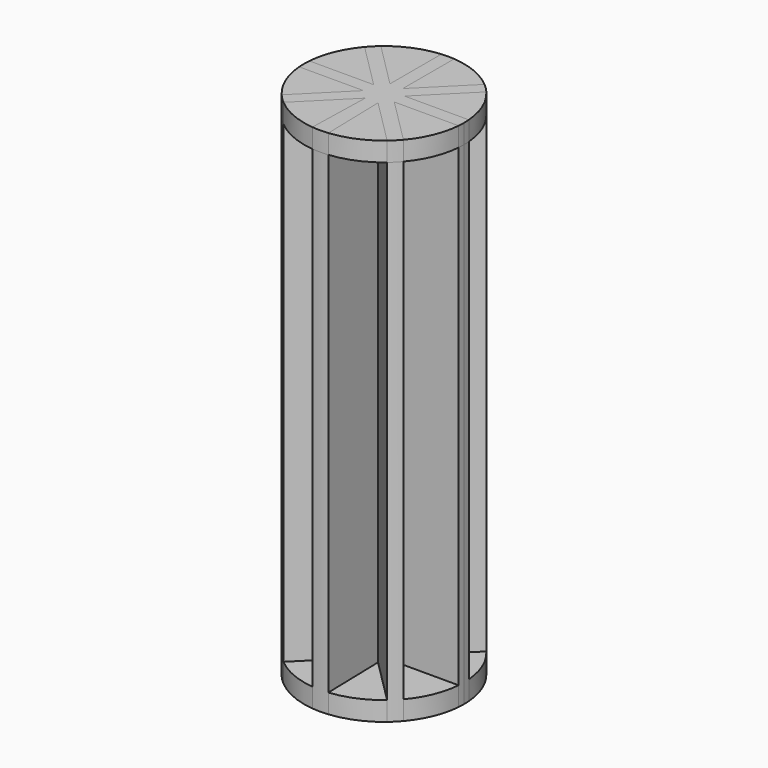
from build123d import *
from build123d import SkipClean  # not in build123d's __all__

# Parameters (mm, degrees)
F1_DEPTH = 3
F2_DEPTH = 80
F4_DEPTH = 3


with BuildPart() as f1:
    # F0 (on Top) → F1 (new body)
    with BuildSketch(Plane.XY):
        with BuildLine():
            Line((1, 2.4142135624), (8.1033983122, 9.5176118745))
            ThreePointArc((8.1033983122, 9.5176118745), (4.7835429046, 11.5484941564), (1, 12.4599357944))
            Line((1, 12.4599357944), (1, 2.4142135624))
        make_face()
    extrude(amount=F1_DEPTH)



with BuildPart() as f1b:
    # F0 (on Top) → F1, piece 2 (new body)
    with BuildSketch(Plane.XY):
        with BuildLine():
            Line((-1, 2.4142135624), (-1, 12.4599357944))
            ThreePointArc((-1, 12.4599357944), (-4.7835429046, 11.5484941564), (-8.1033983122, 9.5176118745))
            Line((-8.1033983122, 9.5176118745), (-1, 2.4142135624))
        make_face()
    extrude(amount=F1_DEPTH)


with BuildPart() as f1c:
    # F0 (on Top) → F1, piece 3 (new body)
    with BuildSketch(Plane.XY):
        with BuildLine():
            Line((2.4142135624, 1), (12.4599357944, 1))
            ThreePointArc((12.4599357944, 1), (11.5484941564, 4.7835429046), (9.5176118745, 8.1033983122))
            Line((9.5176118745, 8.1033983122), (2.4142135624, 1))
        make_face()
    extrude(amount=F1_DEPTH)


with BuildPart() as f1d:
    # F0 (on Top) → F1, piece 4 (new body)
    with BuildSketch(Plane.XY):
        with BuildLine():
            ThreePointArc((9.5176118745, -8.1033983122), (11.5484941564, -4.7835429046), (12.4599357944, -1))
            Line((12.4599357944, -1), (2.4142135624, -1))
            Line((2.4142135624, -1), (9.5176118745, -8.1033983122))
        make_face()
    extrude(amount=F1_DEPTH)


with BuildPart() as f1e:
    # F0 (on Top) → F1, piece 5 (new body)
    with BuildSketch(Plane.XY):
        with BuildLine():
            Line((-12.4599357944, 1), (-2.4142135624, 1))
            Line((-2.4142135624, 1), (-9.5176118745, 8.1033983122))
            ThreePointArc((-9.5176118745, 8.1033983122), (-11.5484941564, 4.7835429046), (-12.4599357944, 1))
        make_face()
    extrude(amount=F1_DEPTH)


with BuildPart() as f1f:
    # F0 (on Top) → F1, piece 6 (new body)
    with BuildSketch(Plane.XY):
        with BuildLine():
            ThreePointArc((-12.4599357944, -1), (-11.5484941564, -4.7835429046), (-9.5176118745, -8.1033983122))
            Line((-9.5176118745, -8.1033983122), (-2.4142135624, -1))
            Line((-2.4142135624, -1), (-12.4599357944, -1))
        make_face()
    extrude(amount=F1_DEPTH)


with BuildPart() as f1g:
    # F0 (on Top) → F1, piece 7 (new body)
    with BuildSketch(Plane.XY):
        with BuildLine():
            ThreePointArc((-8.1033983122, -9.5176118745), (-4.899257332, -11.499881634), (-1.25, -12.4373429638))
            Line((-1.25, -12.4373429638), (-1, -2.4142135624))
            Line((-1, -2.4142135624), (-8.1033983122, -9.5176118745))
        make_face()
    extrude(amount=F1_DEPTH)


with BuildPart() as f1h:
    # F0 (on Top) → F1, piece 8 (new body)
    with BuildSketch(Plane.XY):
        with BuildLine():
            ThreePointArc((1.25, -12.4373429638), (4.899257332, -11.499881634), (8.1033983122, -9.5176118745))
            Line((8.1033983122, -9.5176118745), (1, -2.4142135624))
            Line((1, -2.4142135624), (1.25, -12.4373429638))
        make_face()
    extrude(amount=F1_DEPTH)


with BuildPart() as f1_1:
    add(f1.part, clean=False)

    add(f1b.part)  # F2 merges F1b

    add(f1c.part)  # F2 merges F1c

    add(f1d.part)  # F2 merges F1d

    add(f1e.part)  # F2 merges F1e

    add(f1f.part)  # F2 merges F1f

    add(f1g.part)  # F2 merges F1g

    add(f1h.part)  # F2 merges F1h
    # F0 (on Top) → F2 (join)
    with BuildSketch(Plane.XY):
        with BuildLine():
            Line((1, 2.4142135624), (1, 12.4599357944))
            ThreePointArc((1, 12.4599357944), (0, 12.5), (-1, 12.4599357944))
            Line((-1, 12.4599357944), (-1, 2.4142135624))
            Line((-1, 2.4142135624), (0, 1.4142135624))
            Line((0, 1.4142135624), (1, 2.4142135624))
        make_face()
        with BuildLine():
            Line((2.4142135624, 1), (9.5176118745, 8.1033983122))
            ThreePointArc((9.5176118745, 8.1033983122), (8.8388347648, 8.8388347648), (8.1033983122, 9.5176118745))
            Line((8.1033983122, 9.5176118745), (1, 2.4142135624))
            Line((1, 2.4142135624), (0, 1.4142135624))
            Line((0, 1.4142135624), (-1, 2.4142135624))
            Line((-1, 2.4142135624), (-8.1033983122, 9.5176118745))
            ThreePointArc((-8.1033983122, 9.5176118745), (-8.8388347648, 8.8388347648), (-9.5176118745, 8.1033983122))
            Line((-9.5176118745, 8.1033983122), (-2.4142135624, 1))
            Line((-2.4142135624, 1), (0, -1.4142135624))
            Line((0, -1.4142135624), (1, -2.4142135624))
            Line((1, -2.4142135624), (8.1033983122, -9.5176118745))
            ThreePointArc((8.1033983122, -9.5176118745), (8.8388347648, -8.8388347648), (9.5176118745, -8.1033983122))
            Line((9.5176118745, -8.1033983122), (2.4142135624, -1))
            Line((2.4142135624, -1), (1.4142135624, 0))
            Line((1.4142135624, 0), (2.4142135624, 1))
        make_face()
        with BuildLine():
            Line((-1, -2.4142135624), (0, -1.4142135624))
            Line((0, -1.4142135624), (-2.4142135624, 1))
            Line((-2.4142135624, 1), (-12.4599357944, 1))
            ThreePointArc((-12.4599357944, 1), (-12.5, 0), (-12.4599357944, -1))
            Line((-12.4599357944, -1), (-2.4142135624, -1))
            Line((-2.4142135624, -1), (-9.5176118745, -8.1033983122))
            ThreePointArc((-9.5176118745, -8.1033983122), (-8.8388347648, -8.8388347648), (-8.1033983122, -9.5176118745))
            Line((-8.1033983122, -9.5176118745), (-1, -2.4142135624))
        make_face()
        with BuildLine():
            ThreePointArc((12.4599357944, -1), (12.4899799325, -0.5004011242), (12.5, 0))
            ThreePointArc((12.5, 0), (12.4899799325, 0.5004011242), (12.4599357944, 1))
            Line((12.4599357944, 1), (2.4142135624, 1))
            Line((2.4142135624, 1), (1.4142135624, 0))
            Line((1.4142135624, 0), (2.4142135624, -1))
            Line((2.4142135624, -1), (12.4599357944, -1))
        make_face()
        with BuildLine():
            ThreePointArc((-1.25, -12.4373429638), (0, -12.5), (1.25, -12.4373429638))
            Line((1.25, -12.4373429638), (1, -2.4142135624))
            Line((1, -2.4142135624), (0, -1.4142135624))
            Line((0, -1.4142135624), (-1, -2.4142135624))
            Line((-1, -2.4142135624), (-1.25, -12.4373429638))
        make_face()
    extrude(amount=F2_DEPTH)

    # F3 (on face) → F4 (join)
    with BuildSketch(Plane.XY.offset(80)):
        with BuildLine():
            Line((1, 2.4142135624), (8.1033983122, 9.5176118745))
            ThreePointArc((8.1033983122, 9.5176118745), (4.7835429046, 11.5484941564), (1, 12.4599357944))
            Line((1, 12.4599357944), (1, 2.4142135624))
        make_face()
        with BuildLine():
            Line((-1, 2.4142135624), (-1, 12.4599357944))
            ThreePointArc((-1, 12.4599357944), (-4.7835429046, 11.5484941564), (-8.1033983122, 9.5176118745))
            Line((-8.1033983122, 9.5176118745), (-1, 2.4142135624))
        make_face()
        with BuildLine():
            ThreePointArc((12.4599357944, -1), (12.4899799325, -0.5004011242), (12.5, 0))
            ThreePointArc((12.5, 0), (12.4899799325, 0.5004011242), (12.4599357944, 1))
            Line((12.4599357944, 1), (2.4142135624, 1))
            Line((2.4142135624, 1), (9.5176118745, 8.1033983122))
            ThreePointArc((9.5176118745, 8.1033983122), (8.8388347648, 8.8388347648), (8.1033983122, 9.5176118745))
            Line((8.1033983122, 9.5176118745), (1, 2.4142135624))
            Line((1, 2.4142135624), (1, 12.4599357944))
            ThreePointArc((1, 12.4599357944), (0, 12.5), (-1, 12.4599357944))
            Line((-1, 12.4599357944), (-1, 2.4142135624))
            Line((-1, 2.4142135624), (-8.1033983122, 9.5176118745))
            ThreePointArc((-8.1033983122, 9.5176118745), (-8.8388347648, 8.8388347648), (-9.5176118745, 8.1033983122))
            Line((-9.5176118745, 8.1033983122), (-2.4142135624, 1))
            Line((-2.4142135624, 1), (-12.4599357944, 1))
            ThreePointArc((-12.4599357944, 1), (-12.5, 0), (-12.4599357944, -1))
            Line((-12.4599357944, -1), (-2.4142135624, -1))
            Line((-2.4142135624, -1), (-9.5176118745, -8.1033983122))
            ThreePointArc((-9.5176118745, -8.1033983122), (-8.8388347648, -8.8388347648), (-8.1033983122, -9.5176118745))
            Line((-8.1033983122, -9.5176118745), (-1, -2.4142135624))
            Line((-1, -2.4142135624), (-1.25, -12.4373429638))
            ThreePointArc((-1.25, -12.4373429638), (0, -12.5), (1.25, -12.4373429638))
            Line((1.25, -12.4373429638), (1, -2.4142135624))
            Line((1, -2.4142135624), (8.1033983122, -9.5176118745))
            ThreePointArc((8.1033983122, -9.5176118745), (8.8388347648, -8.8388347648), (9.5176118745, -8.1033983122))
            Line((9.5176118745, -8.1033983122), (2.4142135624, -1))
            Line((2.4142135624, -1), (12.4599357944, -1))
        make_face()
        with BuildLine():
            Line((-2.4142135624, 1), (-9.5176118745, 8.1033983122))
            ThreePointArc((-9.5176118745, 8.1033983122), (-11.5484941564, 4.7835429046), (-12.4599357944, 1))
            Line((-12.4599357944, 1), (-2.4142135624, 1))
        make_face()
        with BuildLine():
            ThreePointArc((-12.4599357944, -1), (-11.5484941564, -4.7835429046), (-9.5176118745, -8.1033983122))
            Line((-9.5176118745, -8.1033983122), (-2.4142135624, -1))
            Line((-2.4142135624, -1), (-12.4599357944, -1))
        make_face()
        with BuildLine():
            ThreePointArc((-8.1033983122, -9.5176118745), (-4.899257332, -11.499881634), (-1.25, -12.4373429638))
            Line((-1.25, -12.4373429638), (-1, -2.4142135624))
            Line((-1, -2.4142135624), (-8.1033983122, -9.5176118745))
        make_face()
        with BuildLine():
            ThreePointArc((1.25, -12.4373429638), (4.899257332, -11.499881634), (8.1033983122, -9.5176118745))
            Line((8.1033983122, -9.5176118745), (1, -2.4142135624))
            Line((1, -2.4142135624), (1.25, -12.4373429638))
        make_face()
        with BuildLine():
            ThreePointArc((9.5176118745, -8.1033983122), (11.5484941564, -4.7835429046), (12.4599357944, -1))
            Line((12.4599357944, -1), (2.4142135624, -1))
            Line((2.4142135624, -1), (9.5176118745, -8.1033983122))
        make_face()
        with BuildLine():
            Line((2.4142135624, 1), (12.4599357944, 1))
            ThreePointArc((12.4599357944, 1), (11.5484941564, 4.7835429046), (9.5176118745, 8.1033983122))
            Line((9.5176118745, 8.1033983122), (2.4142135624, 1))
        make_face()
    with SkipClean():  # cleaning this boolean's faces spoils the solid; the shape is the same uncleaned
        extrude(amount=-F4_DEPTH)


solid = f1_1.part
